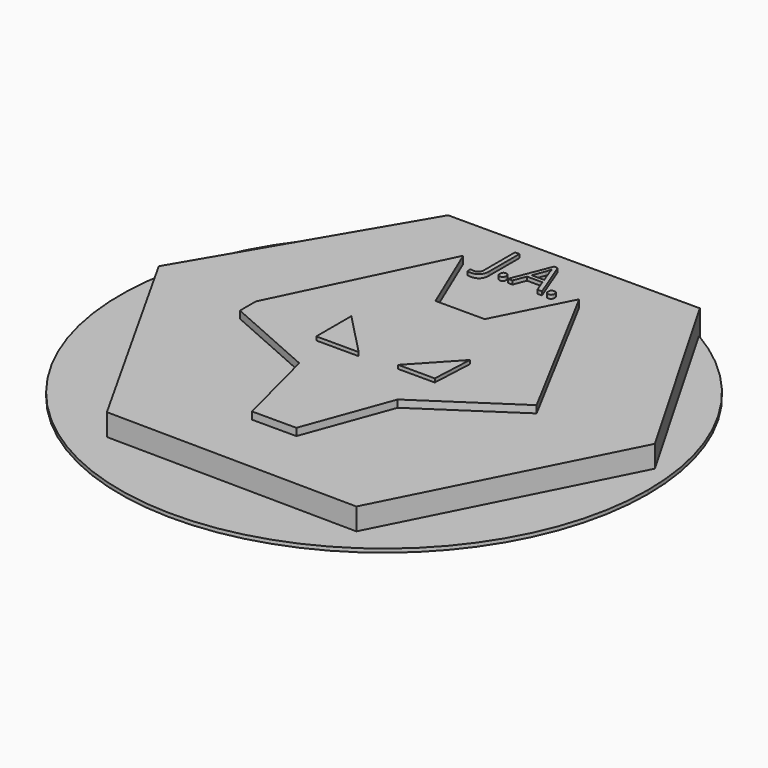
from build123d import *

# Parameters (mm, degrees)
F1_DEPTH     = 7
F2_R         = 72.2889401
F3_DEPTH     = 1
F4_DEPTH     = 2
F5_TEXT_SIZE = 14.7248359604
F6_DEPTH     = 1
F7_DEPTH     = 8


# Not quite as in the source:
# - Text() gives the source's letters only with a copy of the font that has no kerning and outlines rounded to 1/6400 em; it was checked with that copy


with BuildPart() as f1:
    # F0 (on Top) → F1 (new body)
    with BuildSketch(Plane.XY):
        Polygon((35.5432070792, 59.855286032), (-33.4135676965, 59.855286032), (-66.9903531671, 2.7747482527), (-33.4291122854, -56.9484084845), (35.5432070792, -57.7411949635), (67.2554131571, 4.8175734087), align=None)
        Polygon((-53.5130053759, 0), (-25.7655214518, 47.1707247198), (27.086827904, 47.1418075125), (53.9016218932, 0), (27.086827904, -45.5851517618), (-27.879614383, -45.5851517618), align=None, mode=Mode.SUBTRACT)
        Polygon((27.086827904, 47.1418075125), (-25.7655214518, 47.1707247198), (-53.5130053759, 0), (-27.879614383, -45.5851517618), (27.086827904, -45.5851517618), (53.9016218932, 0), align=None)
        Polygon((-38.1858237088, 0), (-16.7806223035, 44.2638471723), (-8.3242459223, 24.1799503565), (5.1531046629, 24.1799503565), (15.1950521395, 43.9995825291), (38.7143492699, 0), (13.8737428933, -16.5163595229), (5.1531046629, -40.2999185026), (-7.0029371418, -40.2999185026), (-13.0809573457, -16.5163595229), (-38.1858237088, -5.4173660465), align=None, mode=Mode.SUBTRACT)
    extrude(amount=F1_DEPTH)

    # F2 (on Top) → F3 (join)
    with BuildSketch(Plane.XY):
        with Locations((0, -3.8317954168)):
            Circle(F2_R)
    extrude(amount=F3_DEPTH)

    # F0 (on Top) → F4 (join)
    with BuildSketch(Plane.XY):
        Polygon((15.1646261413, -5.4228436694), (15.7235749066, 5.9458897449), (5.1531046629, -5.4173660465), align=None)
        Polygon((-5.1572915313, -6.0709256185), (-16.7806223035, 5.9458897449), (-16.7806223035, -6.0645661233), align=None)
    extrude(amount=F4_DEPTH)

    # F5 (on face) → F6 (join)
    with BuildSketch(Plane.XY.offset(7)):
        with Locations((-11.6743390681, 43.3816537261)):
            Text('J.A.', F5_TEXT_SIZE, font='Open Sans', text_align=(TextAlign.LEFT, TextAlign.BOTTOM))
    extrude(amount=F6_DEPTH)

    # F7 (add): faces of the model
    f7_faces = [f1.faces().sort_by_distance(p)[0] for p in [
        (-0.5139065962, 3.389311913, 1),
        (-12.9061787127, -2.0632006656, 2),
        (12.0137685703, -1.6314399903, 2),
    ]]
    extrude(f7_faces, amount=F7_DEPTH)


solid = f1.part
